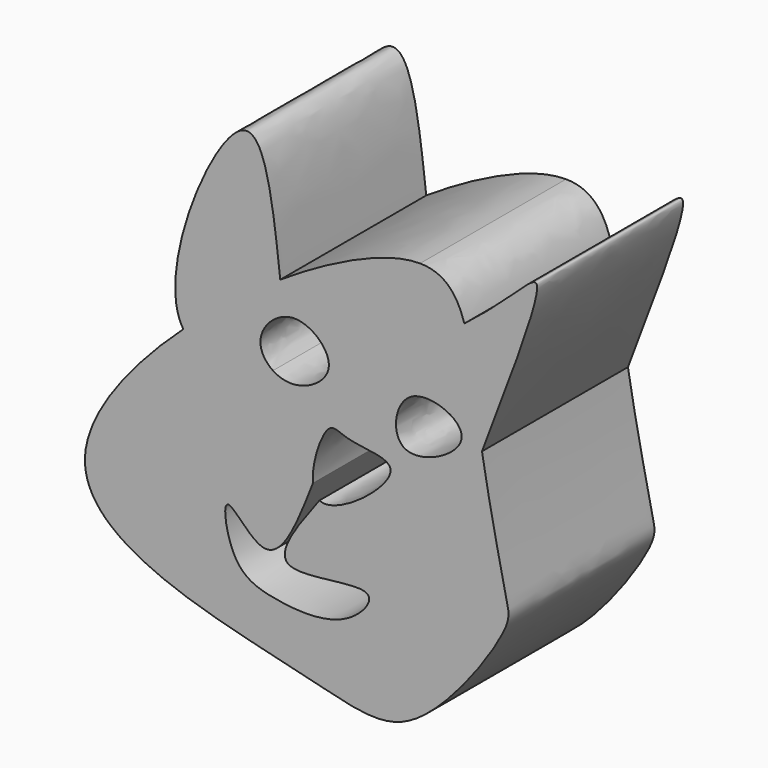
from build123d import *

# Parameters (mm, degrees)
F1_DEPTH = 45.72


with BuildPart() as f1:
    # F0 (on Front) → F1 (new body)
    with BuildSketch(Plane.XZ):
        with BuildLine():
            add(Edge.make_bspline(
                [(43.910749103, 25.2505281901), (42.1388754764, 30.9649923079), (39.0916527947, 34.8205835687), (32.80030936, 34.8858758807)],
                knots=[0.932199267, 0.932199267, 0.932199267, 0.932199267, 1, 1, 1, 1], degree=3))
            add(Edge.make_bspline(
                [(32.80030936, 34.8858758807), (24.7702831742, 34.9692124496), (11.4552672594, 28.8777816348), (-2.2325148238, 19.9122631557)],
                knots=[0, 0, 0, 0, 0.0865382199, 0.0865382199, 0.0865382199, 0.0865382199], degree=3))
            add(Edge.make_bspline(
                [(-2.2325148238, 19.9122631557), (-10.5612558291, 14.4569248885), (-19.0280127082, 7.937461832), (-26.5261184901, 1.0974788287)],
                knots=[0.0865382199, 0.0865382199, 0.0865382199, 0.0865382199, 0.139194992, 0.139194992, 0.139194992, 0.139194992], degree=3))
            add(Edge.make_bspline(
                [(-26.5261184901, 1.0974788287), (-22.9886542385, -4.1322639027), (-14.4170728895, -3.9137787945), (-4.0609406224, -0.7431087672)],
                knots=[0.3881355526, 0.3881355526, 0.3881355526, 0.3881355526, 0.4929988103, 0.4929988103, 0.4929988103, 0.4929988103], degree=3))
            add(Edge.make_bspline(
                [(-4.0609406224, -0.7431087672), (-6.0030433933, 0.5381836069), (-9.4639300434, 6.1031972563), (-2.9866250923, 12.5191974373), (1.3271797216, 12.5134121627)],
                knots=[0.6000611593, 0.6000611593, 0.6000611593, 0.6000611593, 0.7469206026, 1, 1, 1, 1], degree=3))
            add(Edge.make_bspline(
                [(1.3271797216, 12.5134121627), (5.6508481483, 12.5076136599), (10.1904979201, 8.4174011216), (9.9304039713, 4.7399289904)],
                knots=[0, 0, 0, 0, 0.2536580692, 0.2536580692, 0.2536580692, 0.2536580692], degree=3))
            add(Edge.make_bspline(
                [(9.9304039713, 4.7399289904), (22.1722137776, 10.41955143), (34.8807317151, 18.31775117), (43.910749103, 25.2505281901)],
                knots=[0.5377816342, 0.5377816342, 0.5377816342, 0.5377816342, 0.6515086604, 0.6515086604, 0.6515086604, 0.6515086604], degree=3))
        make_face()
        with BuildLine():
            add(Edge.make_bspline(
                [(-2.2325148238, 19.9122631557), (-10.5612558291, 14.4569248885), (-19.0280127082, 7.937461832), (-26.5261184901, 1.0974788287)],
                knots=[0.0865382199, 0.0865382199, 0.0865382199, 0.0865382199, 0.139194992, 0.139194992, 0.139194992, 0.139194992], degree=3))
            add(Edge.make_bspline(
                [(-2.2325148238, 19.9122631557), (-4.0987960003, 36.167044005), (-8.3292168292, 73.0948104563), (-33.8586240841, 11.9377630282), (-26.5261184901, 1.0974788287)],
                knots=[0, 0, 0, 0, 0.1707735189, 0.3881355526, 0.3881355526, 0.3881355526, 0.3881355526], degree=3))
        make_face()
        with BuildLine():
            add(Edge.make_bspline(
                [(43.910749103, 25.2505281901), (55.5891347995, 34.2165844567), (68.6817815124, 51.6345908942), (55.7121653462, 17.9444292517), (48.312171224, -1.5250728335)],
                knots=[0.6515086604, 0.6515086604, 0.6515086604, 0.6515086604, 0.7985901131, 1, 1, 1, 1], degree=3))
            add(Edge.make_bspline(
                [(48.312171224, -1.5250728335), (47.7715190458, 1.6852646187), (46.2851171625, 11.2754123858), (45.3917972357, 20.4740044676), (43.910749103, 25.2505281901)],
                knots=[0.8463914262, 0.8463914262, 0.8463914262, 0.8463914262, 0.8755269696, 0.932199267, 0.932199267, 0.932199267, 0.932199267], degree=3))
        make_face()
        with BuildLine():
            add(Edge.make_bspline(
                [(48.312171224, -1.5250728335), (47.7715190458, 1.6852646187), (46.2851171625, 11.2754123858), (45.3917972357, 20.4740044676), (43.910749103, 25.2505281901)],
                knots=[0.8463914262, 0.8463914262, 0.8463914262, 0.8463914262, 0.8755269696, 0.932199267, 0.932199267, 0.932199267, 0.932199267], degree=3))
            add(Edge.make_bspline(
                [(9.9304039713, 4.7399289904), (22.1722137776, 10.41955143), (34.8807317151, 18.31775117), (43.910749103, 25.2505281901)],
                knots=[0.5377816342, 0.5377816342, 0.5377816342, 0.5377816342, 0.6515086604, 0.6515086604, 0.6515086604, 0.6515086604], degree=3))
            add(Edge.make_bspline(
                [(9.9304039713, 4.7399289904), (9.6652561851, 0.9910005774), (2.6280269785, -3.4564630864), (-2.8996386658, -1.5092717959), (-4.0609406224, -0.7431087672)],
                knots=[0.2536580692, 0.2536580692, 0.2536580692, 0.2536580692, 0.5122449214, 0.6000611593, 0.6000611593, 0.6000611593, 0.6000611593], degree=3))
            add(Edge.make_bspline(
                [(-26.5261184901, 1.0974788287), (-22.9886542385, -4.1322639027), (-14.4170728895, -3.9137787945), (-4.0609406224, -0.7431087672)],
                knots=[0.3881355526, 0.3881355526, 0.3881355526, 0.3881355526, 0.4929988103, 0.4929988103, 0.4929988103, 0.4929988103], degree=3))
            add(Edge.make_bspline(
                [(-26.5261184901, 1.0974788287), (-40.4877162482, -11.6386833624), (-70.3184985819, -50.5967945249), (6.3315811297, -64.6280382988), (30.7525061237, -74.1452326032), (55.9113838372, -38.6481953791), (54.5675388492, -32.4798376177), (50.4538991897, -14.2424348968), (48.312171224, -1.5250728335)],
                knots=[0.139194992, 0.139194992, 0.139194992, 0.139194992, 0.2372427779, 0.4150406984, 0.5358824425, 0.6709306732, 0.7309745084, 0.8463914262, 0.8463914262, 0.8463914262, 0.8463914262], degree=3))
        make_face()
        with BuildLine():
            add(Edge.make_bspline(
                [(5.9506331684, -22.3089876295), (5.5593328026, -18.0702364312), (7.802260478, -11.3157891444), (9.6694547683, -9.2902611941)],
                knots=[0.792941295, 0.792941295, 0.792941295, 0.792941295, 1, 1, 1, 1], degree=3))
            add(Edge.make_bspline(
                [(9.6694547683, -9.2902611941), (11.1204306739, -7.7162459632), (14.1068993186, -10.8431003088), (34.8926951905, -9.9216307194), (11.8493425042, -27.8378942149), (7.5838854536, -25.5956165493)],
                knots=[0, 0, 0, 0, 0.1609030156, 0.3925647705, 0.7172232266, 0.7172232266, 0.7172232266, 0.7172232266], degree=3))
            add(Edge.make_bspline(
                [(7.5838854536, -25.5956165493), (2.0379853151, -32.976269935), (-9.2330320435, -47.9760824551), (25.6820507177, -37.8964653578), (14.0754798837, -52.6680111273), (-4.0366803908, -51.4877121472), (-14.6811508013, -47.6186314295), (-17.8645000463, -27.5523557704), (-4.2583602777, -48.4957650702), (2.1860484699, -31.9742886217), (5.9506331684, -22.3089876295)],
                knots=[0, 0, 0, 0, 0.1396034497, 0.283709296, 0.3791945484, 0.5192773649, 0.6302285533, 0.7380919506, 0.8467878218, 1, 1, 1, 1], degree=3))
        make_face(mode=Mode.SUBTRACT)
        with BuildLine():
            add(Edge.make_bspline(
                [(30.525142327, 4.7399289904), (35.0231218532, 7.2819893708), (52.3345181897, 0.4211629891), (24.4425445133, -13.9490076511), (26.2864261771, 2.3443928779), (30.525142327, 4.7399289904)],
                knots=[0, 0, 0, 0, 0.3303972427, 0.6886468423, 1, 1, 1, 1], degree=3))
        make_face(mode=Mode.SUBTRACT)
    extrude(amount=F1_DEPTH)


solid = f1.part
